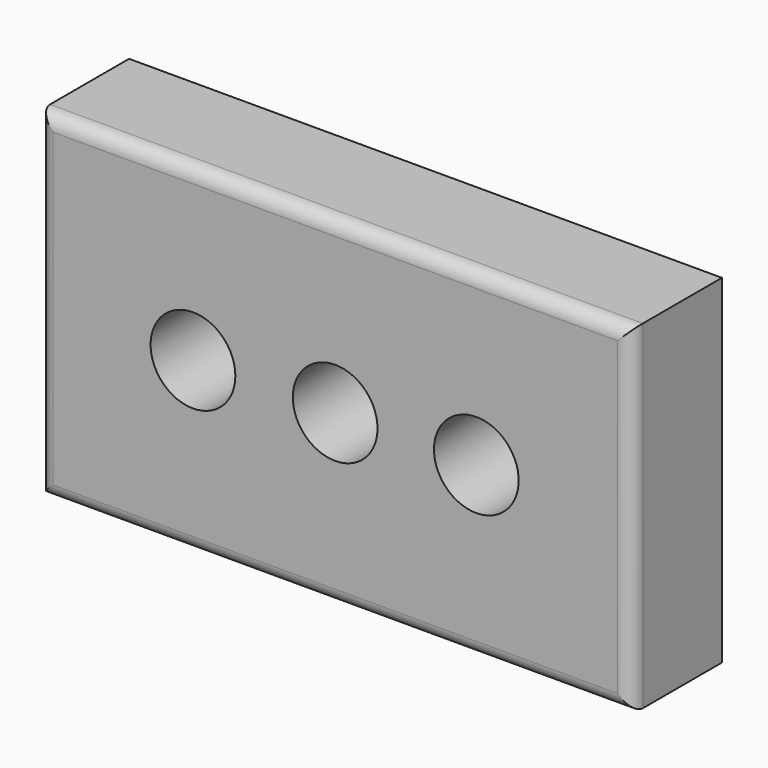
from build123d import *

# Parameters (mm, degrees)
F0_W     = 266.7
F0_H     = 152.4
F0_R     = 19.0629117812
F1_DEPTH = 50.8
F2_DEPTH = 12.7
F3_R     = 6.35


with BuildPart() as f1:
    # F0 (on Front) → F1 (new body)
    with BuildSketch(Plane.XZ):
        Rectangle(F0_W, F0_H)
        with Locations((-63.9682784677, 0)):
            Circle(F0_R, mode=Mode.SUBTRACT)
        with BuildLine():
            ThreePointArc((-19.05, 0), (0, 19.05), (19.05, 0))
            ThreePointArc((19.05, 0), (0, -19.05), (-19.05, 0))
        make_face(mode=Mode.SUBTRACT)
        with BuildLine():
            ThreePointArc((82.55, 0), (63.5, -19.05), (44.45, 0))
            ThreePointArc((44.45, 0), (63.5, 19.05), (82.55, 0))
        make_face(mode=Mode.SUBTRACT)
    extrude(amount=F1_DEPTH)

    # F3
    f3_edges = [f1.edges().sort_by_distance(p)[0] for p in [
        (0, -50.8, 76.2),
        (-133.35, -50.8, 0),
        (133.35, -50.8, 0),
        (0, -50.8, -76.2),
    ]]
    fillet(f3_edges, radius=F3_R)


with BuildPart() as f2:
    # F0 (on Front) → F2 (new body)
    with BuildSketch(Plane.XZ):
        with BuildLine():
            ThreePointArc((-19.05, 0), (0, -19.05), (19.05, 0))
            ThreePointArc((19.05, 0), (0, 19.05), (-19.05, 0))
        make_face()
    extrude(amount=F2_DEPTH)


with BuildPart() as f2b:
    # F0 (on Front) → F2, piece 2 (new body)
    with BuildSketch(Plane.XZ):
        with BuildLine():
            ThreePointArc((82.55, 0), (63.5, 19.05), (44.45, 0))
            ThreePointArc((44.45, 0), (63.5, -19.05), (82.55, 0))
        make_face()
    extrude(amount=F2_DEPTH)


with BuildPart() as f2c:
    # F0 (on Front) → F2, piece 3 (new body)
    with BuildSketch(Plane.XZ):
        with Locations((-63.9682784677, 0)):
            Circle(F0_R)
    extrude(amount=F2_DEPTH)


solid = Compound([f1.part, f2.part, f2b.part, f2c.part])
